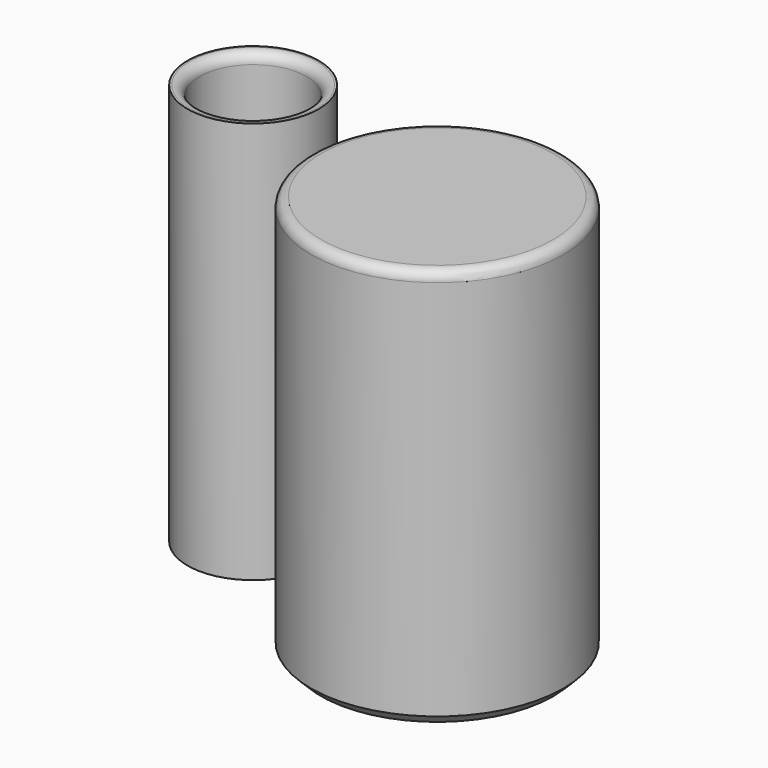
from build123d import *

# Parameters (mm, degrees)
F0_R      = 33.1450146476
F0_R_2    = 27.048974118
F1_DEPTH  = 203.2
F0_R_3    = 63.8478883476
F3_R      = 5.08
F3_2_R    = 5.08
F4_SIZE   = 5.08
F4_2_SIZE = 5.08


# Not quite as in the source:
# - a feature of the source that left no trace in its solid (it failed there, or was rolled back) is left out


with BuildPart() as f1:
    # F0 (on Top) → F1 (new body)
    with BuildSketch(Plane.XY):
        with Locations((-116.4484322071, 29.2191132903)):
            Circle(F0_R)
        with Locations((-116.4484322071, 29.2191132903)):
            Circle(F0_R_2, mode=Mode.SUBTRACT)
    extrude(amount=F1_DEPTH)

    # F3
    f3_edges = [f1.edges().sort_by_distance(p)[0] for p in [
        (-143.497406, 29.219113, 203.2),
    ]]
    fillet(f3_edges, radius=F3_R)

    # F4
    f4_edges = [f1.edges().sort_by_distance(p)[0] for p in [
        (-89.399458, 29.219113, 99.06),
        (-143.497406, 29.219113, 198.12),
        (-143.497406, 29.219113, 0),
    ]]
    chamfer(f4_edges, length=F4_SIZE)


with BuildPart() as f1b:
    # F0 (on Top) → F1, piece 2 (new body)
    with BuildSketch(Plane.XY):
        Circle(F0_R_3)
    extrude(amount=F1_DEPTH)

    # F3#2
    f3_2_edges = [f1b.edges().sort_by_distance(p)[0] for p in [
        (-63.847888, 0, 203.2),
    ]]
    fillet(f3_2_edges, radius=F3_2_R)

    # F4#2
    f4_2_edges = [f1b.edges().sort_by_distance(p)[0] for p in [
        (63.847888, 0, 99.06),
        (-63.847888, 0, 198.12),
        (-63.847888, 0, 0),
    ]]
    chamfer(f4_2_edges, length=F4_2_SIZE)


solid = Compound([f1.part, f1b.part])
